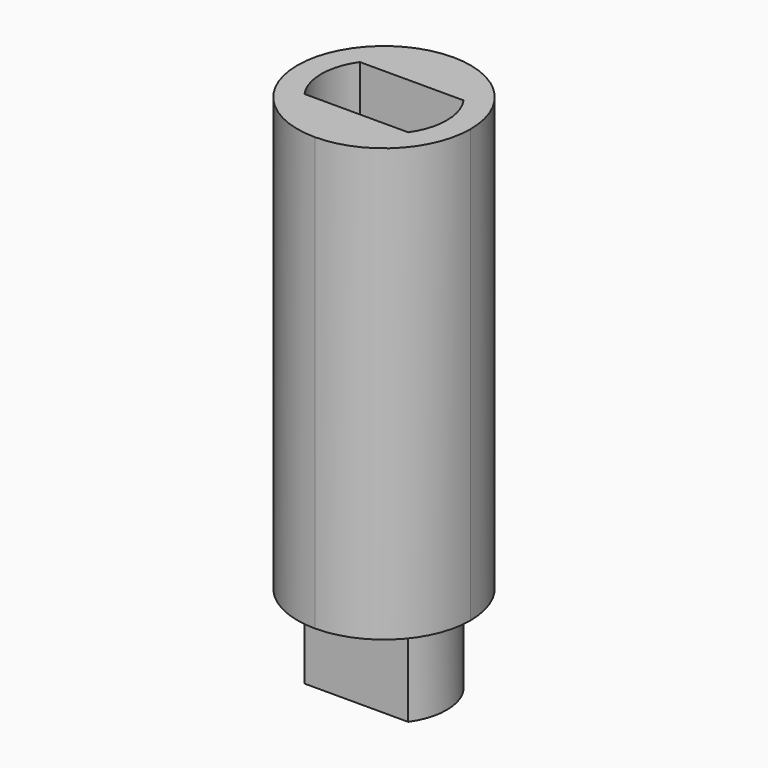
from build123d import *

# Parameters (mm, degrees)
F0_W     = 10
F0_H     = 10
F1_DEPTH = 25
F2_R     = 4.99999
F0_W_2   = 6
F0_H_2   = 4
F3_DEPTH = 5


# Not quite as in the source:
# - a fillet or chamfer is up to 0.001 mm smaller than in the source, because OpenCascade refuses the exact size


with BuildPart() as f1:
    # F0 (on Top) → F1 (new body)
    with BuildSketch(Plane.XY):
        with Locations((-42.5899140537, -34.680514973)):
            Rectangle(F0_W, F0_H)
        with BuildLine():
            ThreePointArc((-45.5899140537, -36.680514973), (-46.2176327304, -34.680514973), (-45.5899140537, -32.680514973))
            Line((-45.5899140537, -32.680514973), (-39.5899140537, -32.680514973))
            ThreePointArc((-39.5899140537, -32.680514973), (-38.9621953769, -34.680514973), (-39.5899140537, -36.680514973))
            Line((-39.5899140537, -36.680514973), (-45.5899140537, -36.680514973))
        make_face(mode=Mode.SUBTRACT)
    extrude(amount=F1_DEPTH)

    # F2 (radius 5 in the source; OpenCascade refuses exactly that, so slightly less here)
    f2_edges = [f1.edges().sort_by_distance(p)[0] for p in [
        (-37.589914, -39.680515, 12.5),
        (-37.589914, -29.680515, 12.5),
        (-47.589914, -39.680515, 12.5),
        (-47.589914, -29.680515, 12.5),
    ]]
    fillet(f2_edges, radius=F2_R)

    # F0 (on Top) → F3 (join)
    with BuildSketch(Plane.XY):
        with Locations((-42.5899140537, -34.680514973)):
            Rectangle(F0_W_2, F0_H_2)
        with BuildLine():
            Line((-45.5899140537, -36.680514973), (-45.5899140537, -32.680514973))
            ThreePointArc((-45.5899140537, -32.680514973), (-46.2176327304, -34.680514973), (-45.5899140537, -36.680514973))
        make_face()
        with BuildLine():
            ThreePointArc((-39.5899140537, -36.680514973), (-38.9621953769, -34.680514973), (-39.5899140537, -32.680514973))
            Line((-39.5899140537, -32.680514973), (-39.5899140537, -36.680514973))
        make_face()
    extrude(amount=-F3_DEPTH)


solid = f1.part
